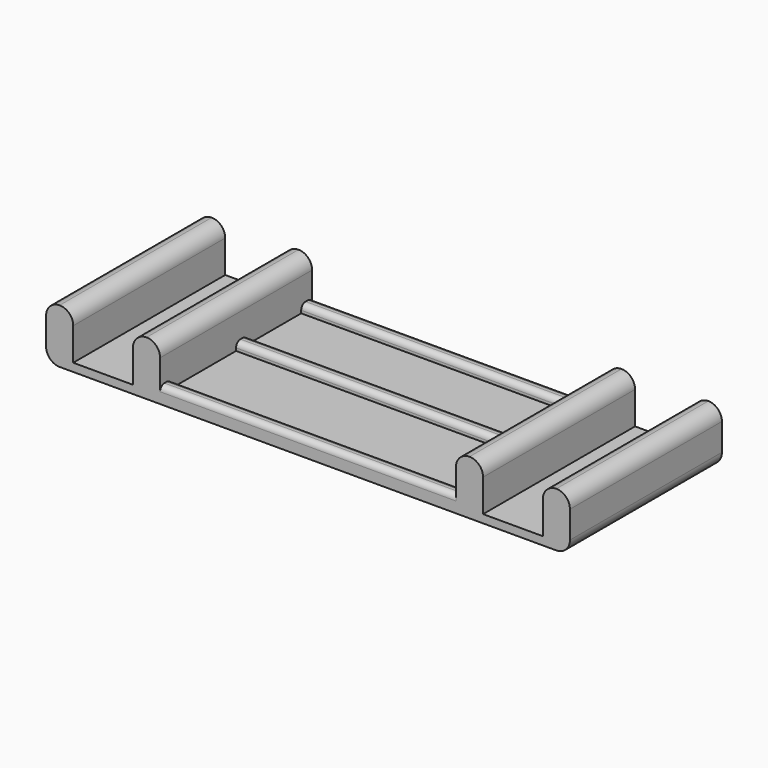
from build123d import *

# Parameters (mm, degrees)
F0_W     = 22
F0_H     = 70
F1_DEPTH = 3
F0_W_2   = 109
F0_H_2   = 25
F0_H_3   = 30
F0_W_3   = 10
F2_DEPTH = 20
F0_H_4   = 5
F3_DEPTH = 6
F4_R     = 4.99999
F5_R     = 5
F6_R     = 2


# Not quite as in the source:
# - a fillet or chamfer is up to 0.001 mm smaller than in the source, because OpenCascade refuses the exact size


with BuildPart() as f1:
    # F0 (on Top) → F1 (new body)
    with BuildSketch(Plane.XY):
        with Locations((-111.672727108, 5)):
            Rectangle(F0_W, F0_H)
    extrude(amount=F1_DEPTH)



with BuildPart() as f1b:
    # F0 (on Top) → F1, piece 2 (new body)
    with BuildSketch(Plane.XY):
        with Locations((39.327272892, 5)):
            Rectangle(F0_W, F0_H)
    extrude(amount=F1_DEPTH)


with BuildPart() as f1c:
    # F0 (on Top) → F1, piece 3 (new body)
    with BuildSketch(Plane.XY):
        with Locations((-36.172727108, 22.5)):
            Rectangle(F0_W_2, F0_H_2)
    extrude(amount=F1_DEPTH)


with BuildPart() as f1d:
    # F0 (on Top) → F1, piece 4 (new body)
    with BuildSketch(Plane.XY):
        with Locations((-36.172727108, -10)):
            Rectangle(F0_W_2, F0_H_3)
    extrude(amount=F1_DEPTH)


with BuildPart() as f1_1:
    add(f1.part)

    add(f1b.part)  # F2 merges F1b

    add(f1c.part)  # F2 merges F1c

    add(f1d.part)  # F2 merges F1d
    # F0 (on Top) → F2 (join)
    with BuildSketch(Plane.XY):
        with Locations((55.327272892, 5)):
            Rectangle(F0_W_3, F0_H)
        with Locations((-127.672727108, 5)):
            Rectangle(F0_W_3, F0_H)
        Polygon((-100.672727108, -30), (-90.672727108, -30), (-90.672727108, -25), (-90.672727108, 5), (-90.672727108, 10), (-90.672727108, 35), (-90.672727108, 40), (-100.672727108, 40), align=None)
        Polygon((18.327272892, -30), (28.327272892, -30), (28.327272892, 40), (18.327272892, 40), (18.327272892, 35), (18.327272892, 10), (18.327272892, 5), (18.327272892, -25), align=None)
    extrude(amount=F2_DEPTH)

    # F0 (on Top) → F3 (join)
    with BuildSketch(Plane.XY):
        with Locations((-36.172727108, 7.5)):
            Rectangle(F0_W_2, F0_H_4)
        with Locations((-36.172727108, -27.5)):
            Rectangle(F0_W_2, F0_H_4)
        with Locations((-36.172727108, 37.5)):
            Rectangle(F0_W_2, F0_H_4)
    extrude(amount=F3_DEPTH)

    # F4 (radius 5 in the source; OpenCascade refuses exactly that, so slightly less here)
    f4_edges = [f1_1.edges().sort_by_distance(p)[0] for p in [
        (50.327273, 5, 20),
        (28.327273, 5, 20),
        (-100.672727, 5, 20),
        (-122.672727, 5, 20),
        (-132.672727, 5, 20),
        (-90.672727, 5, 20),
        (18.327273, 5, 20),
        (60.327273, 5, 20),
    ]]
    fillet(f4_edges, radius=F4_R)

    # F5
    f5_edges = [f1_1.edges().sort_by_distance(p)[0] for p in [
        (-132.672727, 5, 0),
        (60.327273, 5, 0),
    ]]
    fillet(f5_edges, radius=F5_R)

    # F6
    f6_edges = [f1_1.edges().sort_by_distance(p)[0] for p in [
        (-36.172727, 5, 6),
        (-36.172727, 10, 6),
        (-36.172727, -30, 6),
        (-36.172727, 40, 6),
        (-36.172727, 35, 6),
        (-36.172727, -25, 6),
    ]]
    fillet(f6_edges, radius=F6_R)


solid = f1_1.part
